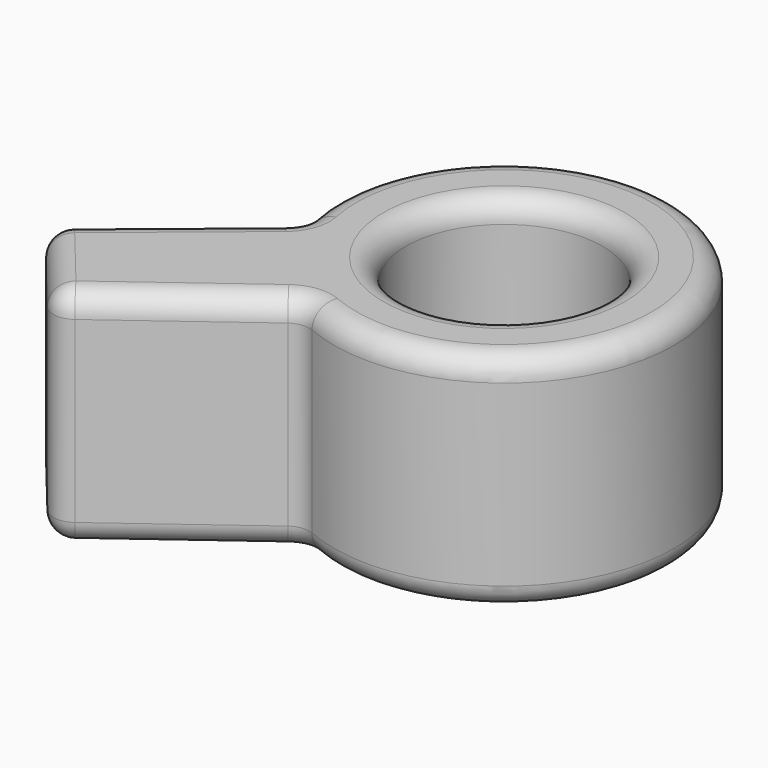
from build123d import *

# Parameters (mm, degrees)
F0_R     = 22.03
F1_DEPTH = 50
F2_R     = 5


with BuildPart() as f1:
    # F0 (on Top) → F1 (new body)
    with BuildSketch(Plane.XY):
        with BuildLine():
            ThreePointArc((19.111431778, -6.8960115293), (56.4366245885, -5.6218490797), (74.7410013376, 26.9318496366))
            ThreePointArc((74.7410013376, 26.9318496366), (31.369006979, 64.6653370911), (0, 16.4892914742))
            ThreePointArc((0, 16.4892914742), (7.1396320987, 2.8221168918), (19.111431778, -6.8960115293))
        make_face()
        with Locations((36.6410013376, 26.9318496366)):
            Circle(F0_R, mode=Mode.SUBTRACT)
        with BuildLine():
            ThreePointArc((19.111431778, -6.8960115293), (7.1396320987, 2.8221168918), (0, 16.4892914742))
            Line((0, 16.4892914742), (-34.7932870747, -12.0488790092))
            Line((-34.7932870747, -12.0488790092), (-17.0362032183, -33.6980354112))
            Line((-17.0362032183, -33.6980354112), (19.111431778, -6.8960115293))
        make_face()
    extrude(amount=F1_DEPTH)

    # F2
    f2_edges = [f1.edges().sort_by_distance(p)[0] for p in [
        (66.142371, 51.041582, 50),
        (14.611001, 26.93185, 50),
        (-17.396644, 2.220206, 50),
        (1.037614, -20.297023, 50),
        (0, 16.489291, 25),
        (-34.793287, -12.048879, 25),
        (19.111432, -6.896012, 25),
        (-17.036203, -33.698035, 25),
        (-25.914745, -22.873457, 0),
        (-25.914745, -22.873457, 50),
        (66.142371, 51.041582, 0),
        (14.611001, 26.93185, 0),
        (-17.396644, 2.220206, 0),
        (1.037614, -20.297023, 0),
    ]]
    fillet(f2_edges, radius=F2_R)


solid = f1.part
